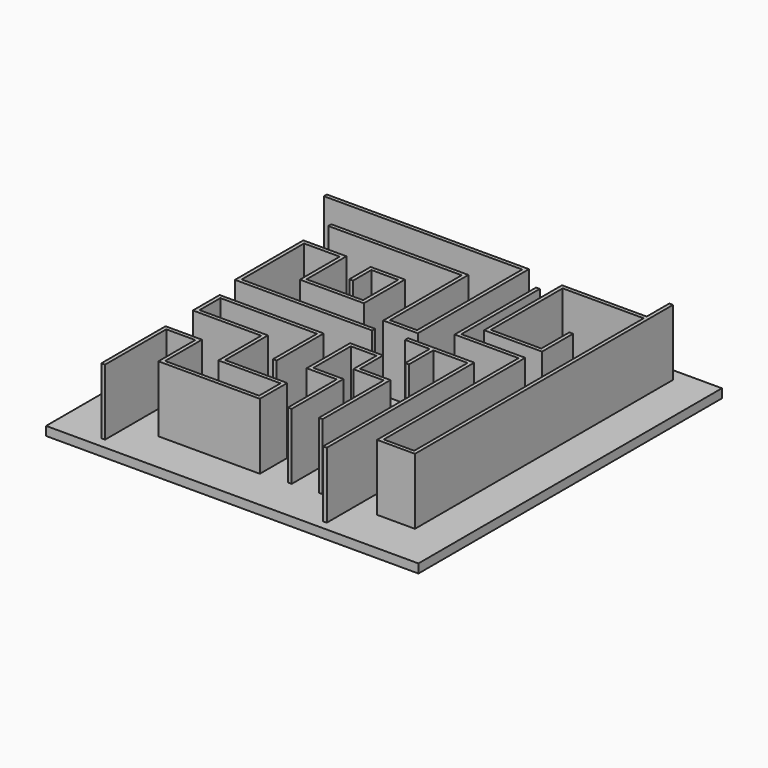
from build123d import *

# Parameters (mm, degrees)
F1_DEPTH = 25.654
F0_W     = 1.2699998915
F0_H     = 10.4394
F0_W_2   = 8.3973463625
F0_H_2   = 1.27
F2_W     = 127.459269017
F2_H     = 129.8603862524
F3_DEPTH = 3.048


# Not quite as in the source:
# - ends of sketch curves that miss each other by under 0.0002 mm in the source are joined
# - the program builds the solid bodies; features that only make, move or delete a surface that nothing else refers to are left out


with BuildPart() as f1:
    # F0 (on Top) → F1 (new body)
    with BuildSketch(Plane.XY):
        Polygon((-44.6478687227, -33.835709095), (-44.6478687227, -61.3113231957), (-43.3778688312, -61.3113231957), (-43.3778688312, -35.1057089865), (-33.4520824254, -35.1057089865), (-33.4520824254, -50.8787445724), (1.2699998915, -50.8787445724), (1.2699998915, -39.1802079976), (-19.9727192521, -39.1802079976), (-19.9727192521, -20.8631325513), (-43.3778688312, -20.8631325513), (-43.3778688312, -11.9549604133), (-10.3013357148, -11.9549604133), (-10.3013357148, -30.7828616351), (-9.0313358232, -30.7828616351), (-9.0313358232, -10.6849605218), (-44.6478687227, -10.6849605218), (-44.6478687227, -22.1331324428), (-21.2427191436, -22.1331324428), (-21.2427191436, -40.4502078891), (0, -40.4502078891), (0, -49.6087446809), (-32.1820825338, -49.6087446809), (-32.1820825338, -33.835709095), align=None)
    extrude(amount=F1_DEPTH)


with BuildPart() as f1b:
    # F0 (on Top) → F1, piece 2 (new body)
    with BuildSketch(Plane.XY):
        Polygon((0, -1.2699998915), (0, 0), (-45.6654839218, 0), (-45.6654839218, 26.7124027014), (-33.4541015327, 26.7124027014), (-33.4541015327, 9.6673453227), (-11.575373821, 9.6673453227), (-11.575373821, 27.2212084383), (-23.2779495418, 27.2212084383), (-23.2779495418, 18.0626716465), (-22.0079496503, 18.0626716465), (-22.0079496503, 25.9512085468), (-12.8453737125, 25.9512085468), (-12.8453737125, 10.9373452142), (-32.1841016412, 10.9373452142), (-32.1841016412, 27.9824025929), (-46.9354838133, 27.9824025929), (-46.9354838133, -1.2699998915), align=None)
    extrude(amount=F1_DEPTH)


with BuildPart() as f1c:
    # F0 (on Top) → F1, piece 3 (new body)
    with BuildSketch(Plane.XY):
        Polygon((0, 6.3681719211), (0, 39.9264097214), (-46.9354838133, 39.9264097214), (-46.9354838133, 38.6564097214), (-1.27, 38.6564097214), (-1.27, 5.0981719211), (10.555739623, 5.0981719211), (10.555739623, 52.6514952838), (-46.670460377, 52.6514952838), (-58.6400814354, 52.6514952838), (-58.6400814354, 52.2722989818), (-58.6400814354, 51.3814952838), (-46.670460377, 51.3814952838), (9.285739623, 51.3814952838), (9.285739623, 6.3681719211), align=None)
    extrude(amount=F1_DEPTH)


with BuildPart() as f1d:
    # F0 (on Top) → F1, piece 4 (new body)
    with BuildSketch(Plane.XY):
        Polygon((31.6732786596, -10.4394), (31.6732786596, -49.6087446809), (31.6732786596, -61.82012707), (32.9432785511, -61.82012707), (32.9432785511, -49.6087446809), (32.9432785511, -10.4394), (32.9432785511, 1.2699998915), (19.9707001448, 1.2699998915), (18.7007002532, 1.2699998915), (18.7007002532, 0), (19.9707001448, 0), (31.6732786596, 0), align=None)
        with Locations((19.335700199, -5.2197)):
            Rectangle(F0_W, F0_H)
        with Locations((14.502027072, 0.635)):
            Rectangle(F0_W_2, F0_H_2)
    extrude(amount=F1_DEPTH)


with BuildPart() as f1e:
    # F0 (on Top) → F1, piece 5 (new body)
    with BuildSketch(Plane.XY):
        Polygon((10.3033538908, -29.2564388365), (10.3033538908, -50.1175522804), (11.5733537823, -50.1175522804), (11.5733537823, -27.9864389449), (1.2699998915, -27.9864389449), (1.2699998915, -11.9549604133), (10.050971061, -11.9549604133), (10.050971061, -21.8767095357), (20.481524989, -21.8767095357), (20.481524989, -49.6087446809), (21.7515248805, -49.6087446809), (21.7515248805, -20.6067096442), (11.3209709525, -20.6067096442), (11.3209709525, -10.6849605218), (0, -10.6849605218), (0, -29.2564388365), align=None)
    extrude(amount=F1_DEPTH)


with BuildPart() as f1f:
    # F0 (on Top) → F1, piece 6 (new body)
    with BuildSketch(Plane.XY):
        Polygon((19.9707001448, 11.9569795206), (19.9707001448, 45.5382876098), (18.7007002532, 45.5382876098), (18.7007002532, 10.6869796291), (40.5794270337, 10.6869796291), (40.5794270337, -49.8611293733), (53.5499863327, -49.8611293733), (53.5499863327, 44.5206686854), (53.5499863327, 60.5481117964), (52.2799864411, 60.5481117964), (52.2799864411, 50.8706686854), (52.2799864411, 49.6006686854), (52.2799864411, -48.5911294818), (41.8494269252, -48.5911294818), (41.8494269252, 11.9569795206), align=None)
        Polygon((24.5580426735, 49.6006686854), (52.2799864411, 49.6006686854), (52.2799864411, 50.8706686854), (23.2880426735, 50.8706686854), (23.2880426735, 17.5639590412), (43.1194269252, 17.5639590412), (43.1194269252, 30.7973590412), (41.8494269252, 30.7973590412), (41.8494269252, 18.8339590412), (24.5580426735, 18.8339590412), align=None)
    extrude(amount=F1_DEPTH)


with BuildPart() as f3:
    # F2 (on Top) → F3 (new body)
    with BuildSketch(Plane.XY):
        with Locations((3.0588377267, 0.0096485019)):
            Rectangle(F2_W, F2_H)
    extrude(amount=F3_DEPTH)


solid = Compound([f1.part, f1b.part, f1c.part, f1d.part, f1e.part, f1f.part, f3.part])
